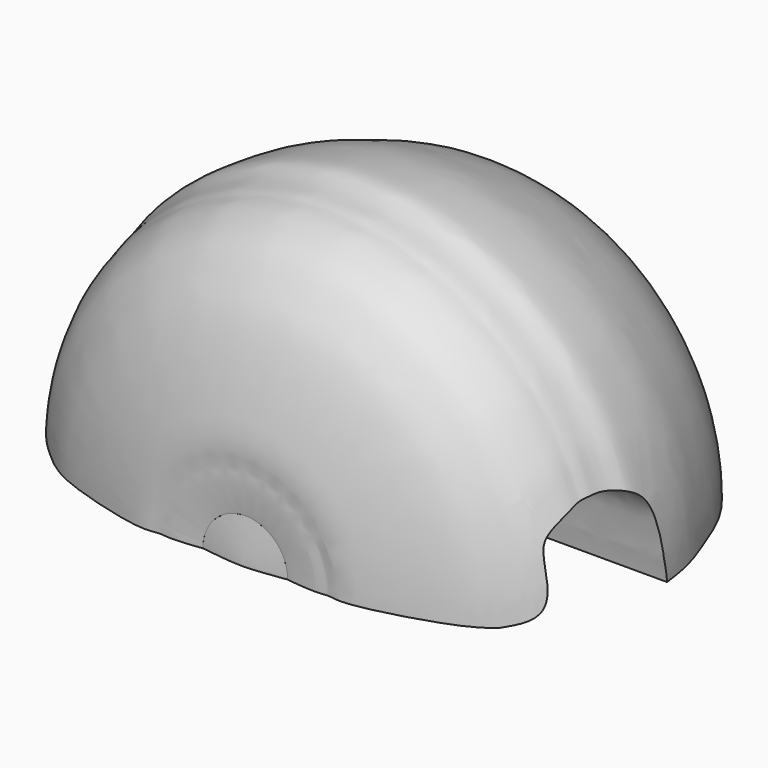
from build123d import *

# Parameters (mm, degrees)
F1_ANGLE_BACK = 90
F1_ANGLE      = 180
F3_DEPTH      = 134.62


# Not quite as in the source:
# - a feature names something its author has since deleted; it is built from what else it names


with BuildPart() as f1:
    # F0 (on Right) → F1 (revolve)
    with BuildSketch(Plane.YZ, mode=Mode.PRIVATE) as f1_sk:
        with BuildLine():
            add(Edge.make_bspline(
                [(25.9693935513, 0), (25.7554495422, -0.9793097444), (25.2968001858, -3.078736533), (21.7148346505, -5.2213793653), (20.6980662352, -6.0068523879), (20.2907323837, -6.3215255688)],
                knots=[0, 0, 0, 0, 0.3438478229, 0.7371348387, 1, 1, 1, 1], degree=3))
            add(Edge.make_bspline(
                [(25.9693935513, 0), (25.594578083, 0.6910542956), (24.088048702, 2.1001370532), (24.531260376, 2.9612781781), (24.1979930295, 5.9705856477), (24.3574789082, 8.6753900891), (23.3899970117, 13.8236234498), (22.9535605586, 18.1968624337), (22.8459832473, 22.9194196813), (22.0041762405, 28.5397955947), (20.9153732211, 32.1691226309), (19.6441141091, 35.9671024144), (16.866383436, 38.5390789392), (14.8150010082, 41.6678871635), (12.3654693146, 43.8757679334), (8.1432623013, 47.1787943901), (2.4065819273, 50.2882973837), (-4.3148605897, 52.7369715209), (-11.6574843244, 55.7552343902), (-21.2445551807, 56.9392519026), (-26.8698043732, 57.4320397338), (-29.2823301618, 56.2857917663), (-32.4849188112, 55.5357288151), (-35.1203136659, 55.3922136991), (-36.8785828777, 54.5679426685), (-39.3412544378, 54.3813596032), (-42.6224874023, 52.8260159012), (-46.2742682905, 50.9484967733), (-49.089741438, 48.3390990975), (-51.2338155304, 45.308235551), (-54.4395387263, 41.182880155), (-57.2718547833, 34.1621335724), (-60.0142100197, 25.0038876877), (-61.8631312506, 16.1694651154), (-60.960244111, 12.9315214186), (-61.5669587564, 10.5415562665), (-61.0474391083, 5.1477113243), (-60.8033659849, 3.3356060849), (-60.791566968, 3.350981744)],
                knots=[0, 0, 0, 0, 0.0219149797, 0.0342187836, 0.0567320893, 0.079729982, 0.1101433914, 0.1386595237, 0.1679993985, 0.199972863, 0.2264117684, 0.252769645, 0.2788798481, 0.3045818401, 0.3288582806, 0.3597317618, 0.3942907157, 0.4301131654, 0.4683487811, 0.5105882593, 0.5418592223, 0.5632687043, 0.5875285536, 0.6093594133, 0.6276823716, 0.6484089107, 0.674043738, 0.7015117234, 0.7275899774, 0.7532919653, 0.7836358168, 0.8204933683, 0.8632552568, 0.9033385232, 0.9266099599, 0.9475716089, 0.9799268807, 0.9958951243, 0.9958951243, 0.9958951243, 0.9958951243], degree=3))
            add(Edge.make_bspline(
                [(-60.791566968, 3.350981744), (-60.9389072927, 2.2994767953), (-61.2518888217, 0.0658613396), (-61.7363713725, -4.1970993715), (-61.7605868281, -5.6860575095), (-61.770491302, -6.2950630672)],
                knots=[0, 0, 0, 0, 0.3445590161, 0.7319150943, 1, 1, 1, 1], degree=3))
            Line((-61.770491302, -6.2950630672), (-54.9727032298, -6.3215255688))
            Line((-54.9727032298, -6.3215255688), (20.2907323837, -6.3215255688))
        make_face()
    revolve(f1_sk.sketch.rotate(Axis((0, -17.340985423, -6.3215255688), (0, 1, 0)), -F1_ANGLE_BACK), axis=Axis((0, -17.340985423, -6.3215255688), (0, 1, 0)), revolution_arc=F1_ANGLE)

    # F2 (on Right) → F3 (cut, symmetric)
    with BuildSketch(Plane.YZ):
        with BuildLine():
            add(Edge.make_bspline(
                [(-55.842757225, -7.3527367786), (-53.1244017477, -6.6587297501), (-48.3744595543, -5.4460505054), (-45.5634397007, -1.5887548083), (-45.7583216061, 5.4675488157), (-45.492955426, 10.1111617546), (-41.3664839817, 13.178868869), (-36.1186310142, 16.0981835838), (-27.6570560359, 14.9596346341), (-22.481328702, 11.3044507189), (-20.8320934561, 5.9406324443), (-20.0973355048, -0.1616185794), (-20.197094063, -1.4010670594), (-18.4896321654, -8.8529674445), (-20.6593195383, -8.4384726016), (-21.4298535138, -8.2912705839)],
                knots=[0, 0, 0, 0, 0.0938009734, 0.1639039504, 0.2531642825, 0.3248472087, 0.3981367118, 0.4810779396, 0.5783227179, 0.6611923824, 0.7422852344, 0.8233105389, 0.8679922509, 0.9531193033, 1, 1, 1, 1], degree=3))
            Line((-55.842757225, -7.3527367786), (-21.4298535138, -8.2912705839))
        make_face()
    extrude(amount=F3_DEPTH, both=True, mode=Mode.SUBTRACT)


solid = f1.part
